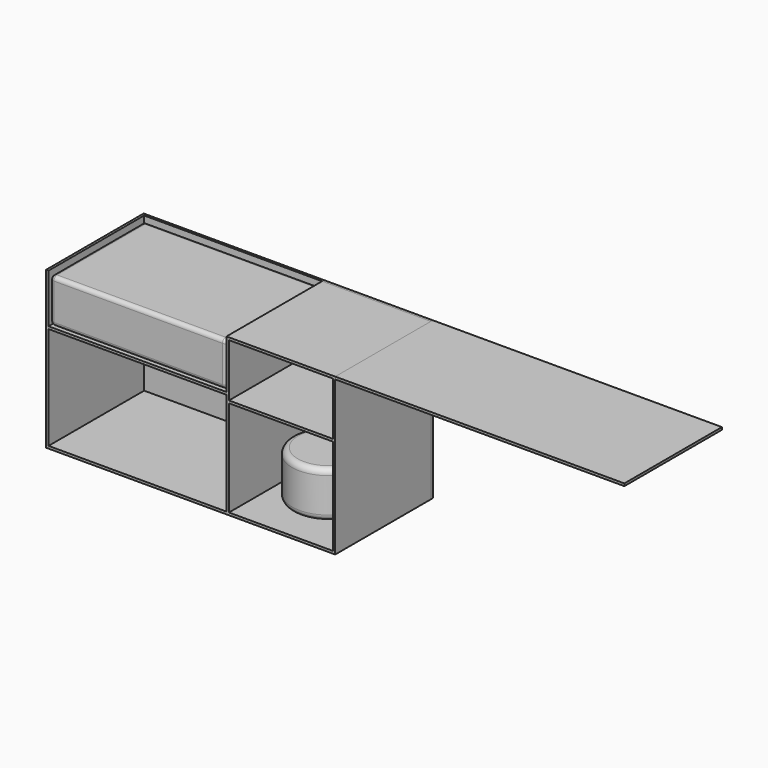
from build123d import *

# Parameters (mm, degrees)
F0_W      = 457.2
F0_H      = 114.3
F1_DEPTH  = 304.8
F2_R      = 10
F3_W      = 461.6222679615
F3_H      = 6.35
F3_W_2    = 269.3277320385
F4_DEPTH  = 310
F5_W      = 269.3277320385
F5_H      = 249.4785221457
F5_W_2    = 461.6222679615
F5_H_2    = 266.7384211302
F5_H_3    = 137.8214778543
F5_H_4    = 126.9115788698
F6_DEPTH  = 6.35
F7_R      = 95
F8_DEPTH  = 120
F9_R      = 15
F11_DEPTH = 6.35


# Not quite as in the source:
# - a length typed as a fraction of an inch, garbled in the dataset ("3 / 203.2 mm" for 3/8 in), is restored


with BuildPart() as f1:
    # F0 (on Front) → F1 (new body)
    with BuildSketch(Plane.XZ):
        with Locations((228.6, 57.15)):
            Rectangle(F0_W, F0_H)
    extrude(amount=F1_DEPTH)

    # F2
    f2_edges = [f1.edges().sort_by_distance(p)[0] for p in [
        (228.6, -304.8, 114.3),
        (0, -304.8, 57.15),
        (228.6, -304.8, 0),
        (457.2, -304.8, 57.15),
        (457.2, -152.4, 114.3),
        (457.2, 0, 57.15),
        (457.2, -152.4, 0),
        (228.6, 0, 114.3),
        (0, -152.4, 114.3),
        (0, -152.4, 0),
        (0, 0, 57.15),
        (228.6, 0, 0),
    ]]
    fillet(f2_edges, radius=F2_R)


with BuildPart() as f4:
    # F3 (on Front) → F4 (new body)
    with BuildSketch(Plane.XZ):
        Polygon((0, 126.9115788698), (-6.35, 126.9115788698), (-6.35, -273.0884211302), (0, -273.0884211302), (0, -6.35), (0, 0), align=None)
        Polygon((0, -273.0884211302), (-6.35, -273.0884211302), (-6.35, -279.4384211302), (743.65, -279.4384211302), (743.65, -273.0884211302), (737.3, -273.0884211302), (467.9722679615, -273.0884211302), (461.6222679615, -273.0884211302), align=None)
        Polygon((737.3, -273.0884211302), (743.65, -273.0884211302), (743.65, 126.9115788698), (737.3, 126.9115788698), (737.3, 120.5615788698), (737.3, -17.2598989844), (737.3, -23.6098989844), align=None)
        Polygon((461.6222679615, 126.9115788698), (461.6222679615, 0), (461.6222679615, -6.35), (461.6222679615, -273.0884211302), (467.9722679615, -273.0884211302), (467.9722679615, -23.6098989844), (467.9722679615, -17.2598989844), (467.9722679615, 120.5615788698), (467.9722679615, 126.9115788698), align=None)
        with Locations((230.8111339808, -3.175)):
            Rectangle(F3_W, F3_H)
        with Locations((602.6361339808, -20.4348989844)):
            Rectangle(F3_W_2, F3_H)
        with Locations((602.6361339808, 123.7365788698)):
            Rectangle(F3_W_2, F3_H)
    extrude(amount=F4_DEPTH)


with BuildPart() as f6:
    # F5 (on face) → F6 (new body)
    with BuildSketch(Plane(origin=(0, 0, 0), x_dir=(-1, 0, 0), z_dir=(0, 1, 0))):
        Polygon((-461.6222679615, 126.9115788698), (-743.65, 126.9115788698), (-743.65, -279.4384211302), (6.35, -279.4384211302), (6.35, 126.9115788698), (0, 126.9115788698), (0, 0), (-461.6222679615, 0), align=None)
        with Locations((-602.6361339808, -148.3491600573)):
            Rectangle(F5_W, F5_H, mode=Mode.SUBTRACT)
        with Locations((-230.8111339808, -139.7192105651)):
            Rectangle(F5_W_2, F5_H_2, mode=Mode.SUBTRACT)
        with Locations((-602.6361339808, 51.6508399427)):
            Rectangle(F5_W, F5_H_3, mode=Mode.SUBTRACT)
        with Locations((-230.8111339808, 63.4557894349)):
            Rectangle(F5_W_2, F5_H_4)
        with Locations((-602.6361339808, 51.6508399427)):
            Rectangle(F5_W, F5_H_3)
        with Locations((-602.6361339808, -148.3491600573)):
            Rectangle(F5_W, F5_H)
        with Locations((-230.8111339808, -139.7192105651)):
            Rectangle(F5_W_2, F5_H_2)
    extrude(amount=F6_DEPTH)


with BuildPart() as f8:
    # F7 (on face) → F8 (new body)
    with BuildSketch(Plane.XY.offset(-273.0884211302)):
        with Locations((591.5974378586, -140.943184495)):
            Circle(F7_R)
    extrude(amount=F8_DEPTH)

    # F9
    f9_edges = [f8.edges().sort_by_distance(p)[0] for p in [
        (496.597438, -140.943184, -153.088421),
        (496.597438, -140.943184, -273.088421),
    ]]
    fillet(f9_edges, radius=F9_R)


with BuildPart() as f11:
    # F10 (on face) → F11 (new body)
    with BuildSketch(Plane.XY.offset(126.9115788698)):
        Polygon((1493.65, 6.35), (743.65, 6.35), (743.65, 0), (743.65, -310), (1493.65, -310), align=None)
    extrude(amount=-F11_DEPTH)


solid = Compound([f1.part, f4.part, f6.part, f8.part, f11.part])
